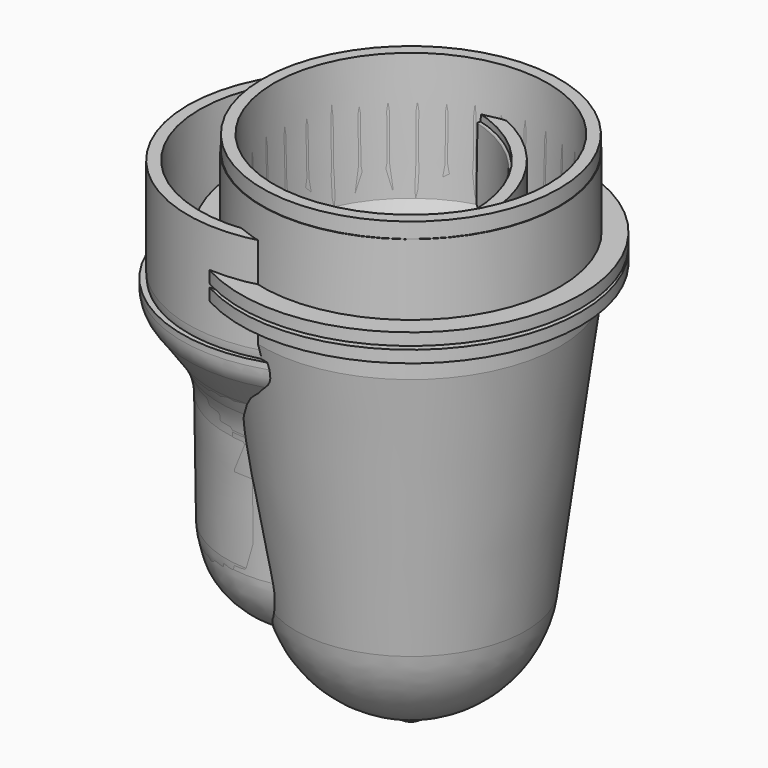
from build123d import *


# Not quite as in the source:
# - ends of sketch curves that miss each other by under 0.0002 mm in the source are joined


with BuildPart() as f1:
    # F0 (on Front) → F1 (revolve)
    with BuildSketch(Plane.XZ):
        with BuildLine():
            Line((8.285, 24.324565), (8.285, 24.325435))
            Line((8.285, 24.325435), (8.285, 24.474565))
            ThreePointArc((8.285, 24.474565), (8.1971320344, 24.6866970344), (7.985, 24.774565))
            Line((7.985, 24.774565), (7.328507, 24.774565))
            ThreePointArc((7.328507, 24.774565), (7.1182343218, 24.6885402341), (7.0285526964, 24.4798010053))
            Line((7.0285526964, 24.4798010053), (6.8227480853, 12.6892282603))
            Line((6.8227480853, 12.6892282603), (6.822464, 12.672953))
            ThreePointArc((6.822464, 12.672953), (6.6564245509, 11.9248810013), (6.2213149313, 11.2941310703))
            Line((6.2213149313, 11.2941310703), (5.613075, 10.699398))
            ThreePointArc((5.613075, 10.699398), (2.6482917301, 6.3776243642), (1.5528098591, 1.2524330021))
            Line((1.5528098591, 1.2524330021), (1.512795, -1.375435))
            Line((1.512795, -1.375435), (1.44158, -12.900045))
            ThreePointArc((1.44158, -12.900045), (0.3773285929, -15.9530813385), (-2.3326028047, -17.7165820889))
            Line((-2.3326028047, -17.7165820889), (-2.3487150182, -17.7206279268))
            Line((-2.3487150182, -17.7206279268), (-4.975, -18.375435))
            Line((-4.975, -18.375435), (-8.975, -18.375435))
            Line((-8.975, -18.375435), (-8.975, -24.774565))
            Line((-8.975, -24.774565), (-7.975, -24.774565))
            Line((-7.975, -24.774565), (-7.093365, -19.774565))
            Line((-7.093365, -19.774565), (-3.873795, -19.753053))
            Line((-3.873795, -19.753053), (-2.570369, -19.476001))
            ThreePointArc((-2.570369, -19.476001), (1.9504213735, -16.7259665821), (3.7656526174, -11.7555370081))
            Line((3.7656526174, -11.7555370081), (3.93795, 1.406243))
            ThreePointArc((3.93795, 1.406243), (4.384698548, 4.0911272277), (5.6136492463, 6.5196798241))
            Line((5.6136492463, 6.5196798241), (8.229902, 10.182328))
            ThreePointArc((8.229902, 10.182328), (8.7841735908, 11.2865899289), (8.975, 12.507326))
            Line((8.975, 12.507326), (8.975, 13.225435))
            Line((8.975, 13.225435), (8.285, 13.225435))
            Line((8.285, 13.225435), (8.285, 24.324565))
        make_face()
    revolve(axis=Axis((-8.975, 0, -21.575), (0, 0, 1)))


with BuildPart() as f3:
    # F2 (on Front) → F3 (revolve)
    with BuildSketch(Plane.XZ):
        with BuildLine():
            Line((8.75, 14.5), (8.75, 25.5))
            Line((8.75, 25.5), (7.375, 25.5))
            Line((7.375, 25.5), (7.081694, 14.29909))
            ThreePointArc((7.081694, 14.29909), (6.8818614226, 13.1511425249), (6.3596729993, 12.1094920005))
            Line((6.3596729993, 12.1094920005), (4.233036, 9.07234))
            ThreePointArc((4.233036, 9.07234), (2.4476875278, 5.4864875736), (1.7931528591, 1.5346030021))
            Line((1.7931528591, 1.5346030021), (1.737795, -2.10087))
            Line((1.737795, -2.10087), (1.66658, -13.625481))
            ThreePointArc((1.66658, -13.625481), (0.6023286685, -16.678517242), (-2.1076025671, -18.4420180288))
            Line((-2.1076025671, -18.4420180288), (-2.1237150182, -18.4460629268))
            Line((-2.1237150182, -18.4460629268), (-4.75, -19.10087))
            Line((-4.75, -19.10087), (-8.75, -19.10087))
            Line((-8.75, -19.10087), (-8.75, -25.5))
            Line((-8.75, -25.5), (-7.75, -25.5))
            Line((-7.75, -25.5), (-6.868365, -20.5))
            Line((-6.868365, -20.5), (-3.648795, -20.478488))
            Line((-3.648795, -20.478488), (-2.345369, -20.201436))
            ThreePointArc((-2.345369, -20.201436), (2.1754217566, -17.4514021153), (3.9906526305, -12.4809720083))
            Line((3.9906526305, -12.4809720083), (4.168737, 1.122926))
            ThreePointArc((4.168737, 1.122926), (4.3942393141, 3.0105426589), (5.0111957953, 4.8086840954))
            Line((5.0111957953, 4.8086840954), (8.187847, 11.621034))
            ThreePointArc((8.187847, 11.621034), (8.6077761114, 12.858105626), (8.75, 14.156743))
            Line((8.75, 14.156743), (8.75, 14.5))
        make_face()
    revolve(axis=Axis((-8.75, 0, -22.300435), (0, 0, 1)))


with BuildPart() as f5:
    # F4 (on Front) → F5 (revolve)
    with BuildSketch(Plane.XZ):
        with BuildLine():
            Line((0, -23.462578), (1, -23.462578))
            Line((1, -23.462578), (1.881635, -18.462578))
            Line((1.881635, -18.462578), (5.101205, -18.441066))
            Line((5.101205, -18.441066), (6.404631, -18.164015))
            ThreePointArc((6.404631, -18.164015), (10.9254213735, -15.4139805821), (12.7406526174, -10.4435510081))
            Line((12.7406526174, -10.4435510081), (12.918737, 3.160348))
            ThreePointArc((12.918737, 3.160348), (13.1442393141, 5.0479646589), (13.7611957953, 6.8461060954))
            Line((13.7611957953, 6.8461060954), (16.903508, 13.584815))
            Line((16.903508, 13.584815), (17.465661, 16.120525))
            Line((17.465661, 16.120525), (17.465661, 19.430821))
            Line((17.465661, 19.430821), (20.006215, 19.501459))
            Line((20.006215, 19.501459), (20.006215, 20.912839))
            Line((20.006215, 20.912839), (17.465661, 20.912839))
            Line((17.465661, 20.912839), (17.465661, 31.074709))
            Line((17.465661, 31.074709), (17.32473, 31.074709))
            Line((17.32473, 31.074709), (16.759971, 31.074709))
            Line((16.759971, 31.074709), (16.124918, 31.074709))
            Line((16.124918, 31.074709), (15.735083, 16.198462))
            Line((15.735083, 16.198462), (15.013063, 14.008942))
            Line((15.013063, 14.008942), (12.983036, 11.109762))
            ThreePointArc((12.983036, 11.109762), (11.1976875278, 7.5239095736), (10.5431528591, 3.5720250021))
            Line((10.5431528591, 3.5720250021), (10.487795, -0.063448))
            Line((10.487795, -0.063448), (10.41658, -11.588059))
            ThreePointArc((10.41658, -11.588059), (9.3523286685, -14.641095242), (6.6423974329, -16.4045960288))
            Line((6.6423974329, -16.4045960288), (6.6262849818, -16.4086409268))
            Line((6.6262849818, -16.4086409268), (4, -17.063448))
            Line((4, -17.063448), (0, -17.063448))
            Line((0, -17.063448), (0, -23.462578))
        make_face()
    revolve(axis=Axis((0, 0, -20.263013), (0, 0, 1)))


with BuildPart() as f7:
    # F6 (on Front) → F7 (revolve)
    with BuildSketch(Plane.XZ):
        with BuildLine():
            Line((-14.48693, 11.399435), (-14.643245, 11.55575))
            Line((-14.643245, 11.55575), (-15.330184, 12.242689))
            ThreePointArc((-15.330184, 12.242689), (-15.5990227835, 12.6393901782), (-15.7017227956, 13.1074700054))
            Line((-15.7017227956, 13.1074700054), (-16.124918, 29.268643))
            Line((-16.124918, 29.268643), (-16.830609, 29.268643))
            Line((-16.830609, 29.268643), (-17.32473, 29.268643))
            Line((-17.32473, 29.268643), (-17.536299, 29.268643))
            Line((-17.536299, 29.268643), (-17.536299, 19.106773))
            Line((-17.536299, 19.106773), (-17.536299, 17.624755))
            Line((-17.536299, 17.624755), (-17.536299, 14.731356))
            Line((-17.536299, 14.731356), (-13.513562, -16.052687))
            ThreePointArc((-13.513562, -16.052687), (-9.8549129967, -23.7248270288), (-2.3783239168, -27.7681005447))
            ThreePointArc((-2.3783239168, -27.7681005447), (-1.5388742478, -28.2337102441), (-1.1536219867, -29.1129419988))
            Line((-1.1536219867, -29.1129419988), (-1.14, -29.268644))
            Line((-1.14, -29.268644), (0, -29.268644))
            Line((0, -29.268644), (0, -28.319565))
            Line((0, -28.319565), (0, -26.027157))
            ThreePointArc((0, -26.027157), (-7.2434873288, -23.2796279503), (-10.8426436089, -16.4193729526))
            Line((-10.8426436089, -16.4193729526), (-14.124183, 10.654225))
            ThreePointArc((-14.124183, 10.654225), (-14.2430547112, 11.0572540598), (-14.48693, 11.399435))
        make_face()
        Polygon((-17.536299, 17.624755), (-17.536299, 19.106773), (-20.006215, 19.106773), (-20.006215, 17.695393), align=None)
    revolve(axis=Axis((0, 0, -27.6479005), (0, 0, -1)))


solid = Compound([f1.part, f3.part, f5.part, f7.part])
